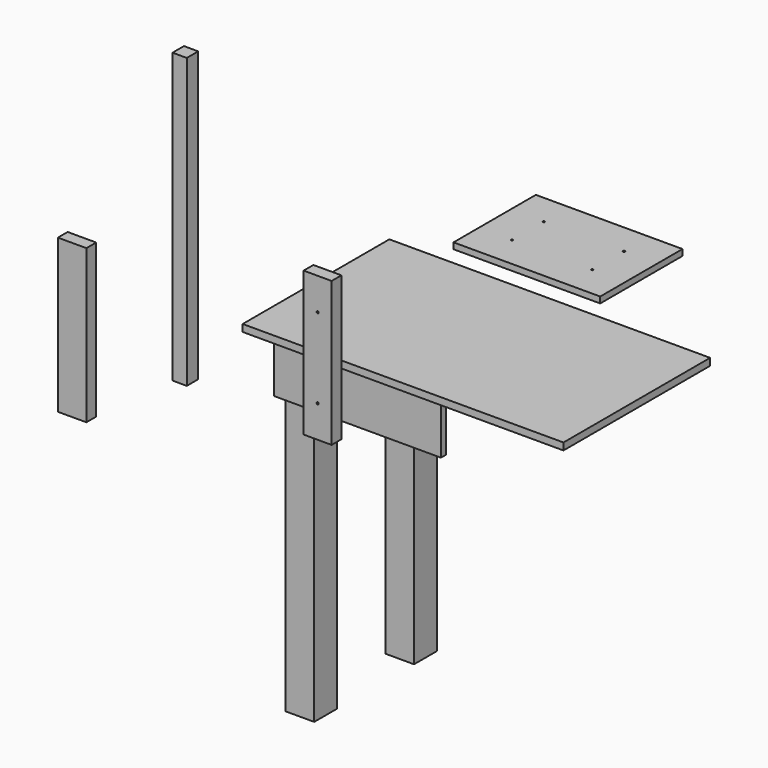
from build123d import *

# Parameters (mm, degrees)
F0_W      = 457.2
F0_H      = 320.675
F1_DEPTH  = 19.05
F2_W      = 1000
F2_H      = 571.5
F3_DEPTH  = 22
F5_DEPTH  = 184
F4_W      = 89
F4_H      = 89
F6_DEPTH  = 1050.925
F7_W      = 44.45
F7_H      = 44.45
F8_DEPTH  = 900
F9_W      = 87.3125
F9_H      = 38.1
F10_DEPTH = 450
F11_R     = 3.175
F12_DEPTH = 19.05
F13_R     = 3.175
F14_DEPTH = 38.1
F15_W     = 88.9
F15_H     = 38.1
F16_DEPTH = 478


# Not quite as in the source:
# - a feature names something its author has since deleted; it is built from what else it names


with BuildPart() as f1:
    # F0 (on Top) → F1 (new body)
    with BuildSketch(Plane.XY):
        with Locations((-95.6145071059, 116.9288526843)):
            Rectangle(F0_W, F0_H)
    extrude(amount=F1_DEPTH)

    # F11 (on face) → F12 (cut, through all)
    with BuildSketch(Plane.XY.offset(19.05)):
        with Locations((29.3854928941, 55.0348526843)):
            Circle(F11_R)
        with Locations((29.3854928941, 178.8228526843)):
            Circle(F11_R)
        with Locations((-220.6145071059, 55.0348526843)):
            Circle(F11_R)
        with Locations((-220.6145071059, 178.8228526843)):
            Circle(F11_R)
    extrude(amount=-F12_DEPTH, mode=Mode.SUBTRACT)


with BuildPart() as f3:
    # F2 (on Top) → F3 (new body)
    with BuildSketch(Plane.XY):
        with Locations((20.9495377159, -385.75)):
            Rectangle(F2_W, F2_H)
    extrude(amount=-F3_DEPTH)

    # F4 (on face) → F5 (join)
    with BuildSketch(Plane(origin=(0, 0, -22), x_dir=(1, 0, 0), z_dir=(0, 0, -1))):
        Polygon((90.9495377159, 611.5), (-409.0504622841, 611.5), (-409.0504622841, 591.5), (-320.0504622841, 591.5), (90.9495377159, 591.5), align=None)
        Polygon((-429.0504622841, 611.5), (-429.0504622841, 100), (-409.0504622841, 100), (-409.0504622841, 113.5), (-409.0504622841, 120), (-409.0504622841, 202.5), (-409.0504622841, 502.5), (-409.0504622841, 591.5), (-409.0504622841, 611.5), align=None)
    extrude(amount=F5_DEPTH)

    # F4 (on face) → F6 (join)
    with BuildSketch(Plane(origin=(0, 0, -22), x_dir=(1, 0, 0), z_dir=(0, 0, -1))):
        with Locations((-364.5504622841, 547)):
            Rectangle(F4_W, F4_H)
        Polygon((-409.0504622841, 120), (-409.0504622841, 113.5), (-320.0504622841, 113.5), (-320.0504622841, 202.5), (-409.0504622841, 202.5), align=None)
    extrude(amount=F6_DEPTH)


with BuildPart() as f8:
    # F7 (on Top) → F8 (new body)
    with BuildSketch(Plane.XY):
        with Locations((-403.6145740495, -989.1184568405)):
            Rectangle(F7_W, F7_H)
    extrude(amount=F8_DEPTH)


with BuildPart() as f10:
    # F9 (on Top) → F10 (new body)
    with BuildSketch(Plane.XY):
        with Locations((44.7211664671, -1015.1306986809)):
            Rectangle(F9_W, F9_H)
    extrude(amount=F10_DEPTH)

    # F13 (on face) → F14 (cut, through all)
    with BuildSketch(Plane.XZ.offset(1034.1806986809)):
        with Locations((44.7211664671, 350)):
            Circle(F13_R)
        with Locations((44.7211664671, 100)):
            Circle(F13_R)
    extrude(amount=-F14_DEPTH, mode=Mode.SUBTRACT)


with BuildPart() as f16:
    # F15 (on Top) → F16 (new body)
    with BuildSketch(Plane.XY):
        with Locations((-496.685385704, -1294.9855373636)):
            Rectangle(F15_W, F15_H)
    extrude(amount=F16_DEPTH)


solid = Compound([f1.part, f3.part, f8.part, f10.part, f16.part])
